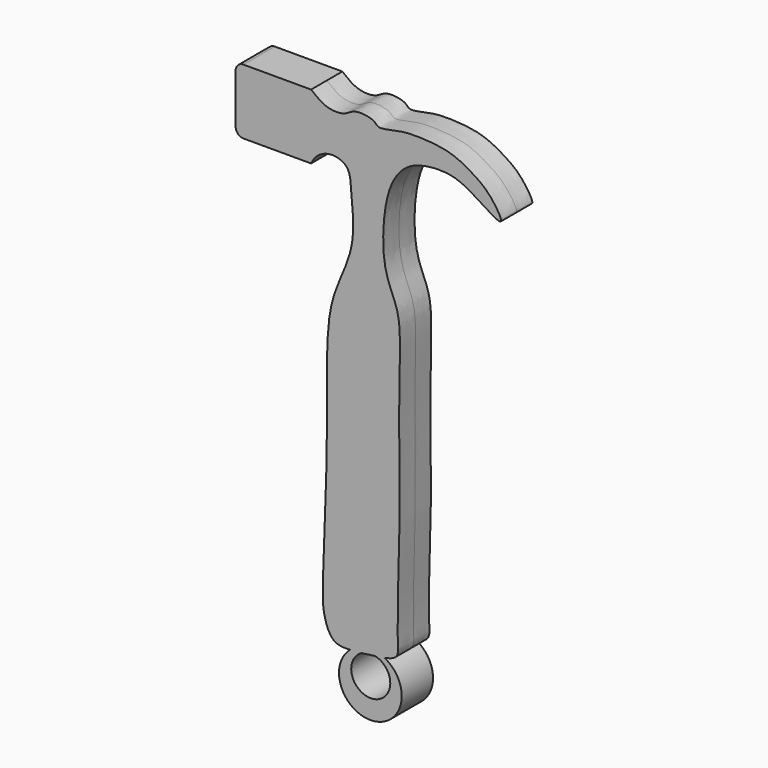
from build123d import *

# Parameters (mm, degrees)
F1_DEPTH = 15.875


with BuildPart() as f1:
    # F0 (on Front) → F1 (new body, symmetric)
    with BuildSketch(Plane.XZ):
        with BuildLine():
            Line((-78.8316577673, 26.8765473738), (-78.8316577673, 79.6747803688))
            Line((-78.8316577673, 79.6747803688), (-133.6865829468, 79.6747803688))
            ThreePointArc((-133.6865829468, 79.6747803688), (-138.1767110073, 77.8149084293), (-140.0365829468, 73.3247803688))
            Line((-140.0365829468, 73.3247803688), (-140.0365829468, 33.2265473738))
            ThreePointArc((-140.0365829468, 33.2265473738), (-138.1767110073, 28.7364193133), (-133.6865829468, 26.8765473738))
            Line((-133.6865829468, 26.8765473738), (-78.8316577673, 26.8765473738))
        make_face()
        with BuildLine():
            add(Edge.make_bspline(
                [(-78.8316577673, 79.6747803688), (-74.867273149, 76.4489380078), (-67.2204041188, 70.2266559627), (-51.859606902, 69.9014743329), (-45.1393060557, 75.9295103171), (-35.5672926956, 76.4212519119), (-26.9719648429, 74.0580519657), (-24.5185923806, 69.2115532847), (-9.7003770976, 73.0818300313), (3.5218065759, 74.7625784338), (32.4342030955, 73.3687633889), (50.6881128796, 63.6555612429), (66.4536668356, 53.3631877885), (82.8183333571, 26.5799982383), (49.2230494452, 51.3433640832), (32.268015648, 56.6936607191), (13.5683150519, 55.8614315402), (-0.7562669832, 51.0880427177), (-13.1076577071, 37.7680178346), (-20.5405945996, 11.8193650544), (-21.0488105396, -27.7193221548), (-11.0826744962, -48.0608105476), (-6.6816315407, -62.3816280735), (-6.6585210267, -87.4077580564), (-7.2309381826, -114.7118704619), (-7.6727435711, -156.602340765), (-6.094526552, -209.2151410636), (-9.836661352, -285.50582649), (-6.9761855518, -303.6062240301), (-14.932897044, -306.0731796427), (-19.3360278675, -306.8922797263)],
                knots=[0, 0, 0, 0, 0.0207823942, 0.0408212762, 0.0564664568, 0.0728580727, 0.0884254163, 0.0994539241, 0.11895194, 0.139651436, 0.1680425501, 0.1923621718, 0.2171481684, 0.2391567759, 0.2672442263, 0.2920082673, 0.3144043704, 0.3349365843, 0.3568480395, 0.384798796, 0.4186125235, 0.4437287799, 0.4641256376, 0.4904639464, 0.5187983252, 0.5527902131, 0.5934456597, 0.6404515436, 0.6612512838, 0.6761906231, 0.6761906231, 0.6761906231, 0.6761906231], degree=3))
            Line((-78.8316577673, 79.6747803688), (-78.8316577673, 26.8765473738))
            add(Edge.make_bspline(
                [(-78.8316577673, 26.8765473738), (-77.022484662, 30.9330394034), (-72.4050763247, 36.0044145501), (-61.8562918517, 39.9147519313), (-47.1640003626, 35.1695972476), (-46.4129918222, 16.4262769767), (-42.116818954, -19.0082345875), (-51.6159275719, -39.2031002217), (-55.4712116718, -48.4385937452)],
                knots=[0, 0, 0, 0, 0.0521369563, 0.1030423593, 0.1585216863, 0.222652622, 0.3162796414, 0.4047795339, 0.4047795339, 0.4047795339, 0.4047795339], degree=3))
            add(Edge.make_bspline(
                [(-64.0298426214, -78.48363373), (-61.812435945, -66.9301917763), (-57.6002283254, -60.298285674), (-55.4712116738, -48.4385937484)],
                knots=[0.8706438085, 0.8706438085, 0.8706438085, 0.8706438085, 0.9006661605, 0.9006661605, 0.9006661605, 0.9006661605], degree=3))
            add(Edge.make_bspline(
                [(-64.0298426151, -78.483633697), (-66.780316687, -98.7430076671), (-65.7695163536, -129.1572469455), (-66.0351291299, -162.7056896687)],
                knots=[0.4923329651, 0.4923329651, 0.4923329651, 0.4923329651, 0.6361102307, 0.6361102307, 0.6361102307, 0.6361102307], degree=3))
            add(Edge.make_bspline(
                [(-66.5412303441, -192.2428831268), (-66.260734863, -182.5165148978), (-66.0656318006, -172.5771027002), (-66.0351291297, -162.7056896114)],
                knots=[0.806596457, 0.806596457, 0.806596457, 0.806596457, 0.8213421237, 0.8213421237, 0.8213421237, 0.8213421237], degree=3))
            add(Edge.make_bspline(
                [(-66.5412303441, -192.2428831268), (-67.2235508932, -219.640667559), (-68.5300791677, -249.5073688179), (-69.2037673306, -267.8069193051), (-69.2628355854, -269.7588843909)],
                knots=[0.6777243549, 0.6777243549, 0.6777243549, 0.6777243549, 0.7934215853, 0.8081974738, 0.8081974738, 0.8081974738, 0.8081974738], degree=3))
            add(Edge.make_bspline(
                [(-68.040415641, -292.0466959732), (-68.9718437312, -285.4449906975), (-69.2992218475, -278.4041660797), (-69.2628355852, -269.7588843999)],
                knots=[0.7375374893, 0.7375374893, 0.7375374893, 0.7375374893, 0.7596414295, 0.7596414295, 0.7596414295, 0.7596414295], degree=3))
            add(Edge.make_bspline(
                [(-68.0404156394, -292.0466959729), (-66.6941727585, -298.4935948833), (-64.1441256006, -305.1380486913), (-60.0192658403, -308.088988082)],
                knots=[0.8771210886, 0.8771210886, 0.8771210886, 0.8771210886, 0.9434612466, 0.9434612466, 0.9434612466, 0.9434612466], degree=3))
            add(Edge.make_bspline(
                [(-47.1750731196, -310.2666801951), (-52.2245748469, -310.3466730848), (-56.7949514606, -309.81148859), (-60.0192658398, -308.0889880767)],
                knots=[0.7013659864, 0.7013659864, 0.7013659864, 0.7013659864, 0.7147892367, 0.7147892367, 0.7147892367, 0.7147892367], degree=3))
            add(Edge.make_bspline(
                [(-37.9094502004, -309.5995166703), (-41.046060424, -309.9578281657), (-44.1940597083, -310.219455758), (-47.1750731196, -310.2666801951)],
                knots=[0.693441464, 0.693441464, 0.693441464, 0.693441464, 0.7013659864, 0.7013659864, 0.7013659864, 0.7013659864], degree=3))
            add(Edge.make_bspline(
                [(-26.9320290536, -308.0889880657), (-30.3665466439, -308.5955665744), (-34.12972936, -309.167739264), (-37.9094502004, -309.5995166703)],
                knots=[0.683892148, 0.683892148, 0.683892148, 0.683892148, 0.693441464, 0.693441464, 0.693441464, 0.693441464], degree=3))
            add(Edge.make_bspline(
                [(-19.3360278675, -306.8922797263), (-21.6059288728, -307.314542016), (-24.1620900798, -307.6804324193), (-26.9320290536, -308.0889880657)],
                knots=[0.6761906231, 0.6761906231, 0.6761906231, 0.6761906231, 0.683892148, 0.683892148, 0.683892148, 0.683892148], degree=3))
        make_face()
        with BuildLine():
            ThreePointArc((-47.1750731196, -310.2666801951), (-27.6349637961, -354.9497222782), (-19.3360278675, -306.8922797263))
            add(Edge.make_bspline(
                [(-19.3360278675, -306.8922797263), (-21.6059288728, -307.314542016), (-24.1620900798, -307.6804324193), (-26.9320290536, -308.0889880657)],
                knots=[0.6761906231, 0.6761906231, 0.6761906231, 0.6761906231, 0.683892148, 0.683892148, 0.683892148, 0.683892148], degree=3))
            ThreePointArc((-26.9320290536, -308.0889880657), (-28.2358224041, -339.2571811148), (-37.9094502004, -309.5995166703))
            add(Edge.make_bspline(
                [(-37.9094502004, -309.5995166703), (-41.046060424, -309.9578281657), (-44.1940597083, -310.219455758), (-47.1750731196, -310.2666801951)],
                knots=[0.693441464, 0.693441464, 0.693441464, 0.693441464, 0.7013659864, 0.7013659864, 0.7013659864, 0.7013659864], degree=3))
        make_face()
        with BuildLine():
            add(Edge.make_bspline(
                [(-60.0192658414, -308.0889880793), (-56.5038321358, -310.603941898), (-51.8445503958, -310.4361516185), (-47.1750731196, -310.2666801951)],
                knots=[0.9434612466, 0.9434612466, 0.9434612466, 0.9434612466, 1, 1, 1, 1], degree=3))
            add(Edge.make_bspline(
                [(-47.1750731196, -310.2666801951), (-52.2245748469, -310.3466730848), (-56.7949514606, -309.81148859), (-60.0192658398, -308.0889880767)],
                knots=[0.7013659864, 0.7013659864, 0.7013659864, 0.7013659864, 0.7147892367, 0.7147892367, 0.7147892367, 0.7147892367], degree=3))
        make_face()
        with BuildLine():
            add(Edge.make_bspline(
                [(-64.0298426214, -78.48363373), (-61.812435945, -66.9301917763), (-57.6002283254, -60.298285674), (-55.4712116738, -48.4385937484)],
                knots=[0.8706438085, 0.8706438085, 0.8706438085, 0.8706438085, 0.9006661605, 0.9006661605, 0.9006661605, 0.9006661605], degree=3))
            add(Edge.make_bspline(
                [(-55.4712116718, -48.4385937452), (-59.2852654764, -57.5753183801), (-62.354936353, -66.146650529), (-64.0298426151, -78.483633697)],
                knots=[0.4047795339, 0.4047795339, 0.4047795339, 0.4047795339, 0.4923329651, 0.4923329651, 0.4923329651, 0.4923329651], degree=3))
        make_face()
        with BuildLine():
            add(Edge.make_bspline(
                [(-69.2628355854, -269.7588843909), (-69.5383653879, -278.8640214351), (-69.4390846946, -285.3487381703), (-68.0404156394, -292.0466959729)],
                knots=[0.8081974738, 0.8081974738, 0.8081974738, 0.8081974738, 0.8771210886, 0.8771210886, 0.8771210886, 0.8771210886], degree=3))
            add(Edge.make_bspline(
                [(-68.040415641, -292.0466959732), (-68.9718437312, -285.4449906975), (-69.2992218475, -278.4041660797), (-69.2628355852, -269.7588843999)],
                knots=[0.7375374893, 0.7375374893, 0.7375374893, 0.7375374893, 0.7596414295, 0.7596414295, 0.7596414295, 0.7596414295], degree=3))
        make_face()
        with BuildLine():
            add(Edge.make_bspline(
                [(-66.5412303441, -192.2428831268), (-66.260734863, -182.5165148978), (-66.0656318006, -172.5771027002), (-66.0351291297, -162.7056896114)],
                knots=[0.806596457, 0.806596457, 0.806596457, 0.806596457, 0.8213421237, 0.8213421237, 0.8213421237, 0.8213421237], degree=3))
            add(Edge.make_bspline(
                [(-66.0351291299, -162.7056896687), (-66.1120066739, -172.4157718366), (-66.2958124373, -182.3884138224), (-66.5412303441, -192.2428831268)],
                knots=[0.6361102307, 0.6361102307, 0.6361102307, 0.6361102307, 0.6777243549, 0.6777243549, 0.6777243549, 0.6777243549], degree=3))
        make_face()
    extrude(amount=F1_DEPTH, both=True)


solid = f1.part
